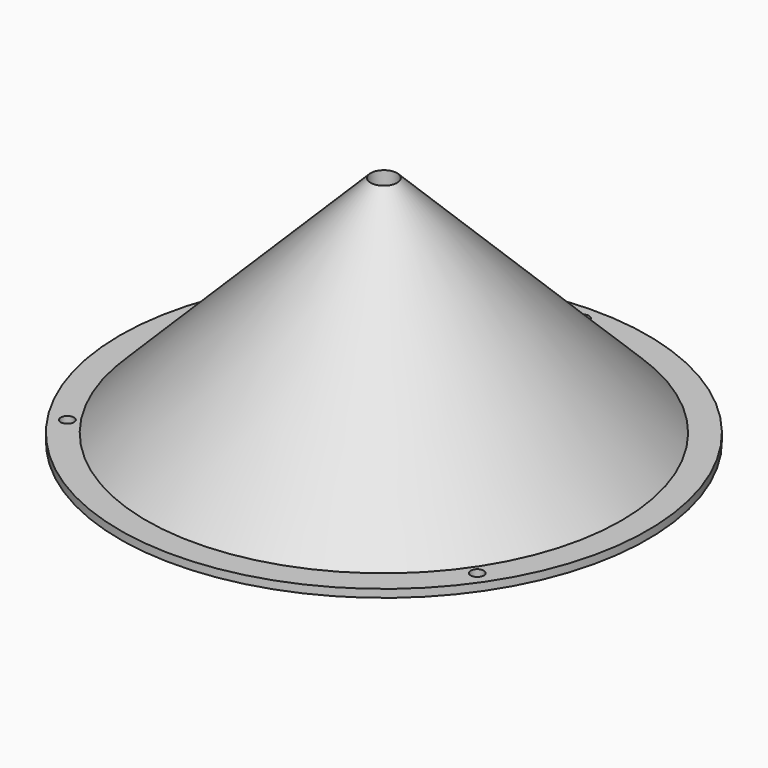
from build123d import *

# Parameters (mm, degrees)
F2_R      = 87
F4_R      = 5
F5_DEPTH  = 93.001
F6_R      = 2.5
F7_DEPTH  = 12.5
F8_R      = 2.5
F9_DEPTH  = 12.5
F10_R     = 2.5
F11_DEPTH = 12.5


# Not quite as in the source:
# - an extrude whose draft closes it to a point is written as a loft to that point


with BuildPart() as f1:
    # F0 (on Front) → F1 (revolve)
    with BuildSketch(Plane.XZ):
        Polygon((-100, 0), (0, 0), (0, 93), (-90, 3), (-100, 3), align=None)
    revolve(axis=Axis((0, 0, 46.5), (0, 0, -1)))

    # F2 (on face) → F3 section 0
    with BuildSketch(Plane(origin=(0, 0, 0), x_dir=(1, 0, 0), z_dir=(0, 0, -1)), mode=Mode.PRIVATE) as f3_s0:
        Circle(F2_R)
    loft([f3_s0.sketch, Vertex(0, 0, 87)], ruled=True, mode=Mode.SUBTRACT)

    # F4 (on Top) → F5 (cut, through all)
    with BuildSketch(Plane.XY):
        Circle(F4_R)
    extrude(amount=F5_DEPTH, mode=Mode.SUBTRACT)

    # F6 (on face) → F7 (cut, symmetric)
    with BuildSketch(Plane.XY.offset(3)):
        with Locations((0, 94)):
            Circle(F6_R)
    extrude(amount=F7_DEPTH, both=True, mode=Mode.SUBTRACT)

    # F8 (on face) → F9 (cut, symmetric)
    with BuildSketch(Plane(origin=(0, 0, 0), x_dir=(1, 0, 0), z_dir=(0, 0, -1))):
        with Locations((-78.3080390386, 51.9985674988)):
            Circle(F8_R)
    extrude(amount=F9_DEPTH, both=True, mode=Mode.SUBTRACT)

    # F10 (on face) → F11 (cut, symmetric)
    with BuildSketch(Plane(origin=(0, 0, 0), x_dir=(1, 0, 0), z_dir=(0, 0, -1))):
        with Locations((77.6980827138, 52.9056513294)):
            Circle(F10_R)
    extrude(amount=F11_DEPTH, both=True, mode=Mode.SUBTRACT)


solid = f1.part
